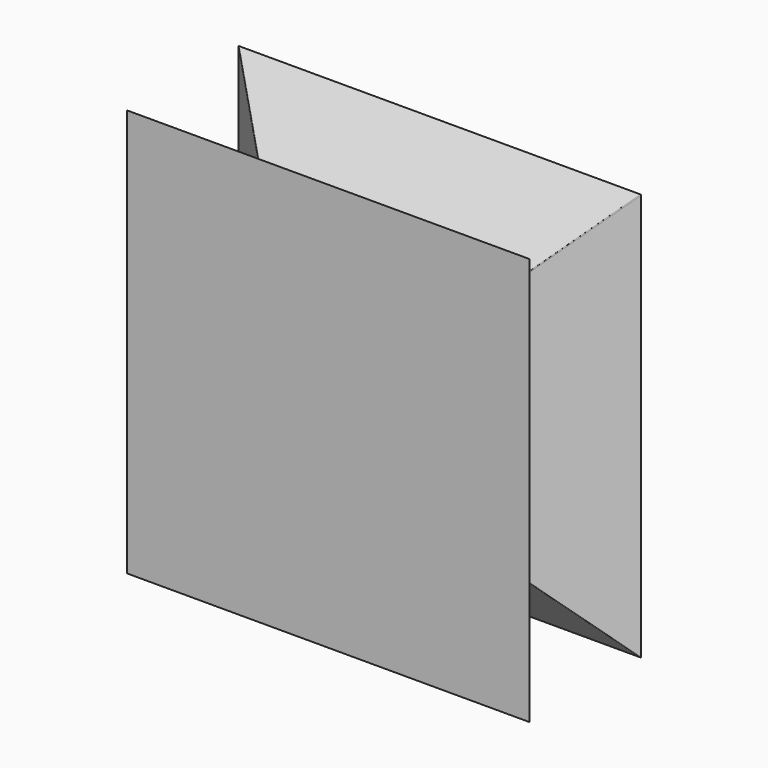
from build123d import *

# Parameters (mm, degrees)
F0_W     = 129.0858983994
F0_H     = 131.8769454956
F1_DEPTH = 38.1
F1_TAPER = -50
F2_R     = 0.508


with BuildPart() as f1:
    # F0 (on Front) → F1 (new body, symmetric)
    with BuildSketch(Plane.XZ):
        Rectangle(F0_W, F0_H)
    extrude(amount=F1_DEPTH, both=True, taper=F1_TAPER)

    # F2
    f2_edges = [f1.edges().sort_by_distance(p)[0] for p in [
        (-87.245855, -19.05, -88.641379),
        (-87.245855, -19.05, 88.641379),
        (-87.245855, 19.05, -88.641379),
        (-87.245855, 19.05, 88.641379),
        (87.245855, -19.05, -88.641379),
        (87.245855, -19.05, 88.641379),
        (87.245855, 19.05, -88.641379),
        (87.245855, 19.05, 88.641379),
    ]]
    fillet(f2_edges, radius=F2_R)


solid = f1.part
